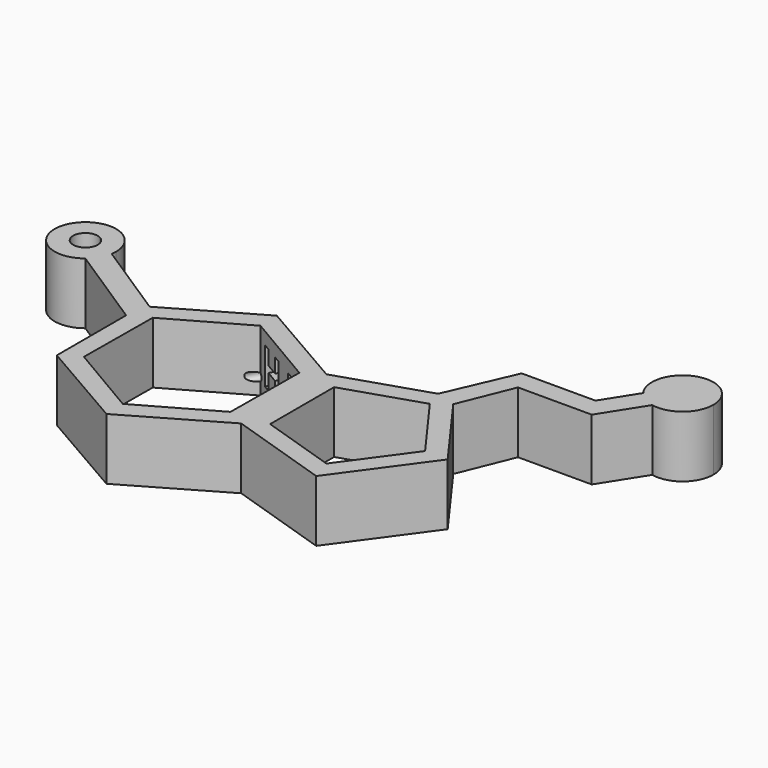
from build123d import *

# Parameters (mm, degrees)
F1_DEPTH     = 5
F2_TEXT_SIZE = 4.1619248903
F3_DEPTH     = 10


# Not quite as in the source:
# - Text() gives the source's letters only with a copy of the font that has no kerning and outlines rounded to 1/6400 em; it was checked with that copy


with BuildPart() as f1:
    # F0 (on Top) → F1 (new body)
    with BuildSketch(Plane.XY):
        with BuildLine():
            ThreePointArc((29.3171706918, 16.3996111482), (26.0204373262, 18.7692558355), (24.8249979366, 14.8892311585))
            ThreePointArc((24.8249979366, 14.8892311585), (25.4800097006, 14.2872663648), (26.3043385711, 13.952775801))
            ThreePointArc((26.3043385711, 13.952775801), (28.3932290185, 14.4589823452), (29.3171706918, 16.3996111482))
        make_face()
        with BuildLine():
            Line((17.103869329, 12.1762663396), (14.7122452344, 6.6735275496))
            Line((14.7122452344, 6.6735275496), (15.7363910355, 7.0062926922))
            Line((15.7363910355, 7.0062926922), (16.3581576661, 6.150504343))
            Line((16.3581576661, 6.150504343), (18.1273650378, 10.5212759227))
            Line((18.1273650378, 10.5212759227), (24.1273650378, 10.5212759227))
            Line((24.1273650378, 10.5212759227), (26.3043385711, 13.952775801))
            ThreePointArc((26.3043385711, 13.952775801), (25.4800097006, 14.2872663648), (24.8249979366, 14.8892311585))
            Line((24.8249979366, 14.8892311585), (23.103869329, 12.1762663396))
            Line((23.103869329, 12.1762663396), (17.103869329, 12.1762663396))
        make_face()
        Polygon((-7.07678584, 4.5744698281), (-7.5, 4.3301270189), (-7.5, 2.7149211333), (-7.5, -4.3301270189), (0, -8.6602540378), (7.5, -4.3301270189), (7.5, 4.3301270189), (0, 8.6602540378), align=None)
        Polygon((-5.9715466473, 3.512923375), (0.0565075606, 6.927972784), (6.028054208, 3.415049409), (5.9715466473, -3.512923375), (-0.0565075606, -6.927972784), (-6.028054208, -3.415049409), align=None, mode=Mode.SUBTRACT)
        Polygon((14.7122452344, 6.6735275496), (7.5, 4.3301270189), (7.5, -4.3301270189), (15.7363910355, -7.0062926922), (20.82676064, 0), (16.3581576661, 6.150504343), (15.7363910355, 7.0062926922), align=None)
        Polygon((8.9866673007, 3.25), (15.1685346566, 5.2586104634), (18.9891387965, 0), (15.1685346566, -5.2586104634), (8.9866673007, -3.25), align=None, mode=Mode.SUBTRACT)
        with BuildLine():
            ThreePointArc((-14.4089840917, 7.2060435767), (-13.8116760704, 7.8939211366), (-13.5004983963, 8.7501459114))
            Line((-13.5004983963, 8.7501459114), (-15.3828863728, 9.973775142))
            ThreePointArc((-15.3828863728, 9.973775142), (-15.0765896624, 9.6180077474), (-14.9663956055, 9.161668637))
            ThreePointArc((-14.9663956055, 9.161668637), (-15.2308290709, 8.4842161492), (-15.8842793519, 8.1650458795))
            Line((-15.8842793519, 8.1650458795), (-14.4089840917, 7.2060435767))
        make_face()
        with BuildLine():
            Line((-15.3828863728, 9.973775142), (-13.5004983963, 8.7501459114))
            ThreePointArc((-13.5004983963, 8.7501459114), (-13.4749358905, 8.9552019605), (-13.4663956055, 9.161668637))
            ThreePointArc((-13.4663956055, 9.161668637), (-18.2184534183, 10.247134255), (-14.4089840917, 7.2060435767))
            Line((-14.4089840917, 7.2060435767), (-15.8842793519, 8.1650458795))
            ThreePointArc((-15.8842793519, 8.1650458795), (-16.9414616206, 9.3835836348), (-15.461065192, 10.0245945743))
            ThreePointArc((-15.461065192, 10.0245945743), (-15.4213831309, 10.0000965722), (-15.3828863728, 9.973775142))
        make_face()
        with BuildLine():
            Line((-7.5, 2.7149211333), (-7.5, 4.3301270189))
            Line((-7.5, 4.3301270189), (-7.07678584, 4.5744698281))
            Line((-7.07678584, 4.5744698281), (-13.5004983963, 8.7501459114))
            ThreePointArc((-13.5004983963, 8.7501459114), (-13.8116760704, 7.8939211366), (-14.4089840917, 7.2060435767))
            Line((-14.4089840917, 7.2060435767), (-7.5, 2.7149211333))
        make_face()
    extrude(amount=F1_DEPTH)

    # F2 (on face) → F3 (cut)
    with BuildSketch(Plane(origin=(3.75, 6.4951905284, 0), x_dir=(-0.8660254038, 0.5, 0), z_dir=(0.5, 0.8660254038, 0))):
        with Locations((-3.7865451272, 1.0304513259)):
            Text('Z.H.', F2_TEXT_SIZE, font='Open Sans', font_style=FontStyle.BOLD, text_align=(TextAlign.LEFT, TextAlign.BOTTOM))
    extrude(amount=-F3_DEPTH, mode=Mode.SUBTRACT)


solid = f1.part
